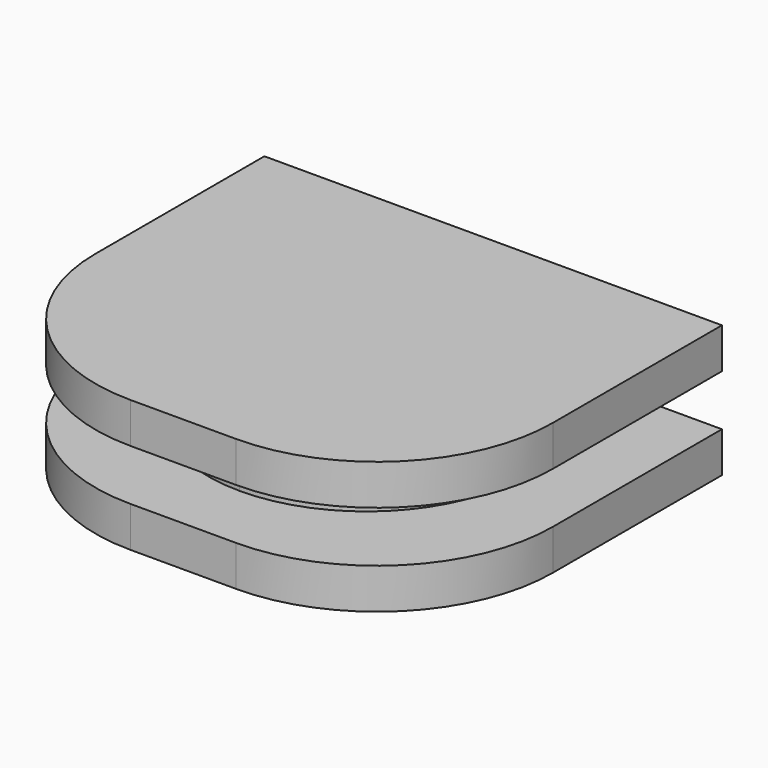
from build123d import *

# Parameters (mm, degrees)
F1_W     = 26
F1_H     = 22
F2_DEPTH = 2.3
F3_START = 5.2
F3_DEPTH = 2.3
F4_START = 2.3
F0_W     = 18
F0_H     = 18
F4_DEPTH = 2.9
F5_R     = 8.99999
F6_R     = 10
F6_2_R   = 10


# Not quite as in the source:
# - a fillet or chamfer is up to 0.001 mm smaller than in the source, because OpenCascade refuses the exact size


with BuildPart() as f2:
    # F1 (on Top) → F2 (new body)
    with BuildSketch(Plane.XY):
        with Locations((0, -2)):
            Rectangle(F1_W, F1_H)
    extrude(amount=F2_DEPTH)

    # F6#2
    f6_2_edges = [f2.edges().sort_by_distance(p)[0] for p in [
        (13, -13, 1.15),
        (-13, -13, 1.15),
    ]]
    fillet(f6_2_edges, radius=F6_2_R)


with BuildPart() as f3:
    # F1 (on Top) → F3 (new body)
    with BuildSketch(Plane.XY.offset(F3_START)):
        with Locations((0, -2)):
            Rectangle(F1_W, F1_H)
    extrude(amount=F3_DEPTH)

    # F6
    f6_edges = [f3.edges().sort_by_distance(p)[0] for p in [
        (-13, -13, 6.35),
        (13, -13, 6.35),
    ]]
    fillet(f6_edges, radius=F6_R)


with BuildPart() as f4:
    # F0 (on Top) → F4 (new body)
    with BuildSketch(Plane.XY.offset(F4_START)):
        Rectangle(F0_W, F0_H)
    extrude(amount=F4_DEPTH)

    # F5 (radius 9 in the source; OpenCascade refuses exactly that, so slightly less here)
    f5_edges = [f4.edges().sort_by_distance(p)[0] for p in [
        (-9, -9, 3.75),
        (9, -9, 3.75),
    ]]
    fillet(f5_edges, radius=F5_R)


solid = Compound([f2.part, f3.part, f4.part])
